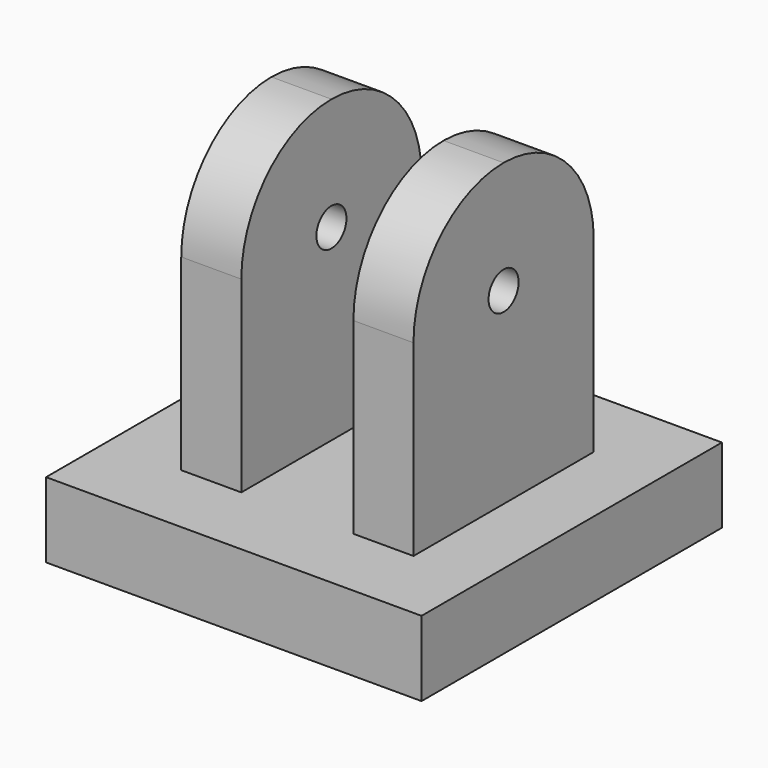
from build123d import *

# Parameters (mm, degrees)
F0_W     = 50
F0_H     = 50
F1_DEPTH = 10
F2_W     = 8
F2_H     = 30
F4_DEPTH = 40
F3_W     = 8
F3_H     = 30
F5_DEPTH = 40
F6_R     = 14.99999
F8_D     = 5


# Not quite as in the source:
# - a fillet or chamfer is up to 0.001 mm smaller than in the source, because OpenCascade refuses the exact size


with BuildPart() as f1:
    # F0 (on Top) → F1 (new body)
    with BuildSketch(Plane.XY):
        with Locations((1.8520187587, -0.2831950238)):
            Rectangle(F0_W, F0_H)
    extrude(amount=F1_DEPTH)

    # F2 (on face) → F4 (join)
    with BuildSketch(Plane.XY.offset(10)):
        with Locations((-9.1479812413, -0.2831950238)):
            Rectangle(F2_W, F2_H)
    extrude(amount=F4_DEPTH)

    # F3 (on face) → F5 (join)
    with BuildSketch(Plane.XY.offset(10)):
        with Locations((13.7779086391, -0.2831950238)):
            Rectangle(F3_W, F3_H)
    extrude(amount=F5_DEPTH)

    # F6 (radius 15 in the source; OpenCascade refuses exactly that, so slightly less here)
    f6_edges = [f1.edges().sort_by_distance(p)[0] for p in [
        (-9.147981, -15.283195, 50),
        (13.777909, -15.283195, 50),
        (-9.147981, 14.716805, 50),
        (13.777909, 14.716805, 50),
    ]]
    fillet(f6_edges, radius=F6_R)

    # F8 (through all)
    with Locations(Plane(origin=(-13.1479812413, 0, 0), x_dir=(0, -1, 0), z_dir=(-1, 0, 0))):
        with Locations((0.2831950238, 35)):
            Hole(F8_D / 2)


solid = f1.part
